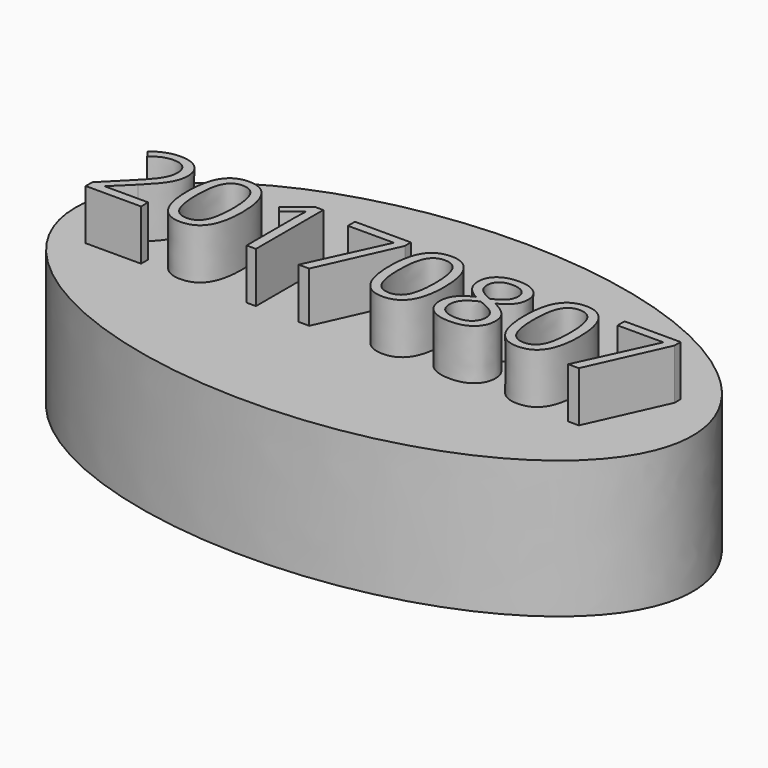
from build123d import *

# Parameters (mm, degrees)
F1_DEPTH     = 32.512
F2_TEXT_SIZE = 27.9245581219
F3_DEPTH     = 11.938


# Not quite as in the source:
# - Text() gives the source's letters only with a copy of the font that has no kerning and outlines rounded to 1/6400 em; it was checked with that copy


with BuildPart() as f1:
    # F0 (on Top) → F1 (new body)
    with BuildSketch(Plane.XY):
        with BuildLine():
            add(Edge.make_bspline(
                [(-73.1115266681, 0), (-73.1115266681, -70.5353604556), (36.555763334, -35.2676802278), (146.2230533361, 0), (36.555763334, 35.2676802278), (-73.1115266681, 70.5353604556), (-73.1115266681, 0)],
                knots=[0, 0, 0, 2.0943951024, 2.0943951024, 4.1887902048, 4.1887902048, 6.2831853072, 6.2831853072, 6.2831853072], degree=2, weights=[1, 0.5, 1, 0.5, 1, 0.5, 1]))
        make_face()
    extrude(amount=F1_DEPTH)

    # F2 (on face) → F3 (join)
    with BuildSketch(Plane.XY.offset(32.512)):
        with Locations((-64.0563184044, -9.9339466542)):
            Text('20170807', F2_TEXT_SIZE, font='Open Sans', text_align=(TextAlign.LEFT, TextAlign.BOTTOM))
    extrude(amount=F3_DEPTH)


solid = f1.part
